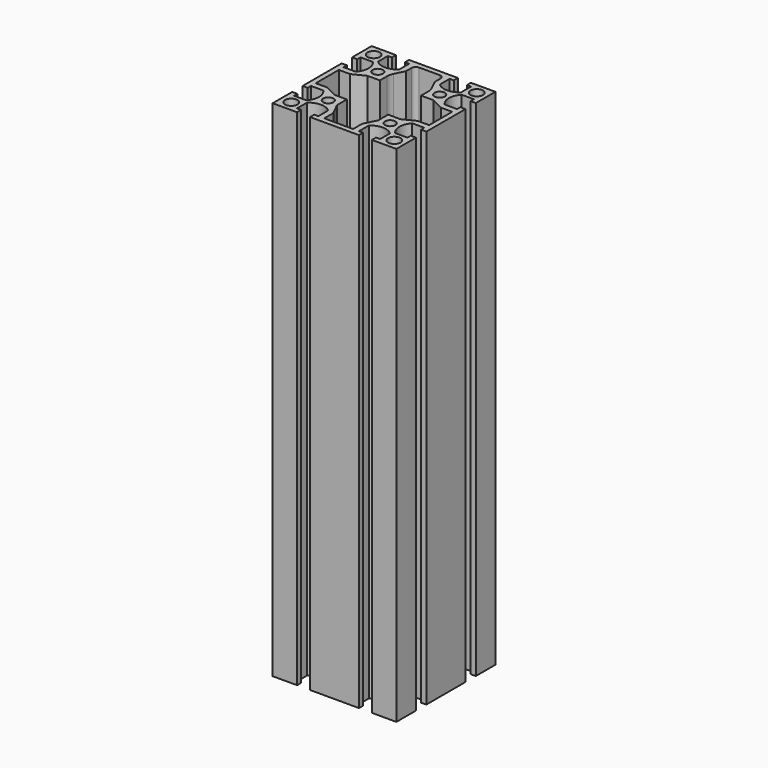
from build123d import *

# Parameters (mm, degrees)
F0_R     = 3
F0_R_2   = 2.5
F1_DEPTH = 244.595
F2_R     = 2
F3_R     = 7


# Not quite as in the source:
# - a feature names something its author has since deleted; it is built from what else it names


with BuildPart() as f1:
    # F0 (on Top) → F1 (new body)
    with BuildSketch(Plane.XY):
        with BuildLine():
            Line((18.15, -30), (30, -30))
            Line((30, -30), (30, -18.15))
            Line((30, -18.15), (27.5, -18.15))
            Line((27.5, -18.15), (27.5, -20.15))
            Line((27.5, -20.15), (21.5477069044, -20.15))
            ThreePointArc((21.5477069044, -20.15), (19.5, -15), (21.5477069044, -9.85))
            Line((21.5477069044, -9.85), (27.5, -9.85))
            Line((27.5, -9.85), (27.5, -11.85))
            Line((27.5, -11.85), (30, -11.85))
            Line((30, -11.85), (30, 11.85))
            Line((30, 11.85), (27.5, 11.85))
            Line((27.5, 11.85), (27.5, 9.85))
            Line((27.5, 9.85), (21.5477069044, 9.85))
            ThreePointArc((21.5477069044, 9.85), (19.5, 15), (21.5477069044, 20.15))
            Line((21.5477069044, 20.15), (27.5, 20.15))
            Line((27.5, 20.15), (27.5, 18.15))
            Line((27.5, 18.15), (30, 18.15))
            Line((30, 18.15), (30, 30))
            Line((30, 30), (18.15, 30))
            Line((18.15, 30), (18.15, 27.5))
            Line((18.15, 27.5), (20.15, 27.5))
            Line((20.15, 27.5), (20.15, 21.5477069044))
            ThreePointArc((20.15, 21.5477069044), (15, 19.5), (9.85, 21.5477069044))
            Line((9.85, 21.5477069044), (9.85, 27.5))
            Line((9.85, 27.5), (11.85, 27.5))
            Line((11.85, 27.5), (11.85, 30))
            Line((11.85, 30), (-11.85, 30))
            Line((-11.85, 30), (-11.85, 27.5))
            Line((-11.85, 27.5), (-9.85, 27.5))
            Line((-9.85, 27.5), (-9.85, 21.5477069044))
            ThreePointArc((-9.85, 21.5477069044), (-15, 19.5), (-20.15, 21.5477069044))
            Line((-20.15, 21.5477069044), (-20.15, 27.5))
            Line((-20.15, 27.5), (-18.15, 27.5))
            Line((-18.15, 27.5), (-18.15, 30))
            Line((-18.15, 30), (-30, 30))
            Line((-30, 30), (-30, 18.15))
            Line((-30, 18.15), (-27.5, 18.15))
            Line((-27.5, 18.15), (-27.5, 20.15))
            Line((-27.5, 20.15), (-21.5477069044, 20.15))
            ThreePointArc((-21.5477069044, 20.15), (-19.5, 15), (-21.5477069044, 9.85))
            Line((-21.5477069044, 9.85), (-27.5, 9.85))
            Line((-27.5, 9.85), (-27.5, 11.85))
            Line((-27.5, 11.85), (-30, 11.85))
            Line((-30, 11.85), (-30, -11.85))
            Line((-30, -11.85), (-27.5, -11.85))
            Line((-27.5, -11.85), (-27.5, -9.85))
            Line((-27.5, -9.85), (-21.5477069044, -9.85))
            ThreePointArc((-21.5477069044, -9.85), (-19.5, -15), (-21.5477069044, -20.15))
            Line((-21.5477069044, -20.15), (-27.5, -20.15))
            Line((-27.5, -20.15), (-27.5, -18.15))
            Line((-27.5, -18.15), (-30, -18.15))
            Line((-30, -18.15), (-30, -30))
            Line((-30, -30), (-18.15, -30))
            Line((-18.15, -30), (-18.15, -27.5))
            Line((-18.15, -27.5), (-20.15, -27.5))
            Line((-20.15, -27.5), (-20.15, -21.5477069044))
            ThreePointArc((-20.15, -21.5477069044), (-15, -19.5), (-9.85, -21.5477069044))
            Line((-9.85, -21.5477069044), (-9.85, -27.5))
            Line((-9.85, -27.5), (-11.85, -27.5))
            Line((-11.85, -27.5), (-11.85, -30))
            Line((-11.85, -30), (11.85, -30))
            Line((11.85, -30), (11.85, -27.5))
            Line((11.85, -27.5), (9.85, -27.5))
            Line((9.85, -27.5), (9.85, -21.5477069044))
            ThreePointArc((9.85, -21.5477069044), (15, -19.5), (20.15, -21.5477069044))
            Line((20.15, -21.5477069044), (20.15, -27.5))
            Line((20.15, -27.5), (18.15, -27.5))
            Line((18.15, -27.5), (18.15, -30))
        make_face()
        with Locations((-25, -25)):
            Circle(F0_R, mode=Mode.SUBTRACT)
        with Locations((-15, -15)):
            Circle(F0_R_2, mode=Mode.SUBTRACT)
        with Locations((25, -25)):
            Circle(F0_R, mode=Mode.SUBTRACT)
        with Locations((15, -15)):
            Circle(F0_R_2, mode=Mode.SUBTRACT)
        with Locations((-25, 25)):
            Circle(F0_R, mode=Mode.SUBTRACT)
        with Locations((-15, 15)):
            Circle(F0_R_2, mode=Mode.SUBTRACT)
        Polygon((-7, 22), (-7, 27.5), (0, 27.5), (7, 27.5), (7, 22), (10, 16), (10, 10), (16, 10), (22, 7), (27.5, 7), (27.5, 0), (27.5, -7), (22, -7), (16, -10), (10, -10), (10, -16), (7, -22), (7, -27.5), (0, -27.5), (-7, -27.5), (-7, -22), (-10, -16), (-10, -10), (-16, -10), (-22, -7), (-27.5, -7), (-27.5, 0), (-27.5, 7), (-22, 7), (-16, 10), (-10, 10), (-10, 16), align=None, mode=Mode.SUBTRACT)
        with Locations((15, 15)):
            Circle(F0_R_2, mode=Mode.SUBTRACT)
        with Locations((25, 25)):
            Circle(F0_R, mode=Mode.SUBTRACT)
    extrude(amount=F1_DEPTH)

    # F2
    f2_edges = [f1.edges().sort_by_distance(p)[0] for p in [
        (-7, 27.5, 122.2975),
        (7, 27.5, 122.2975),
    ]]
    fillet(f2_edges, radius=F2_R)

    # F3
    f3_edges = [f1.edges().sort_by_distance(p)[0] for p in [
        (-10, 16, 122.2975),
        (10, 16, 122.2975),
    ]]
    fillet(f3_edges, radius=F3_R)


solid = f1.part
